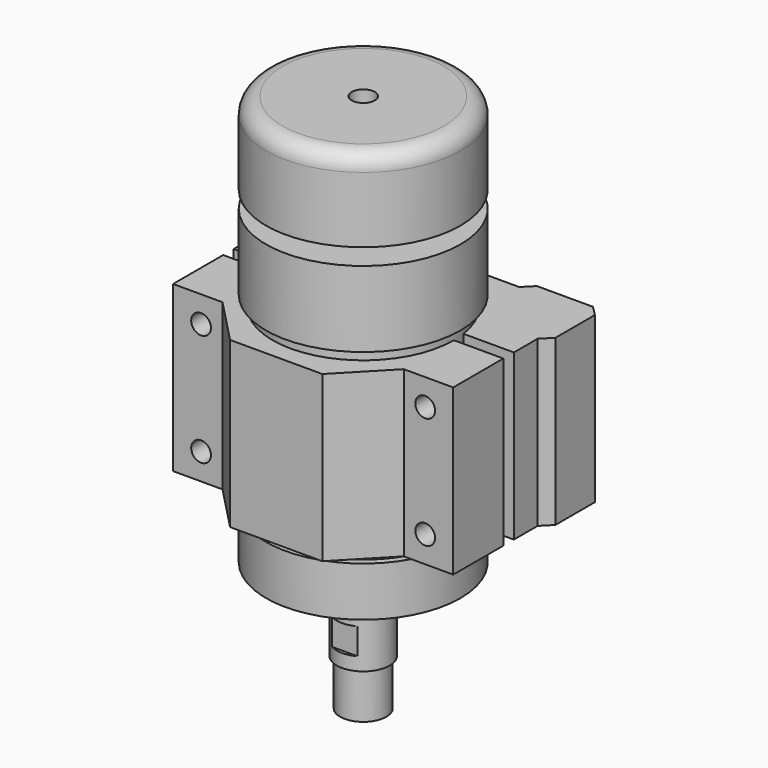
from build123d import *

# Parameters (mm, degrees)
F1_DEPTH      = 28.25
F2_R          = 29.5
F3_DEPTH      = 23
F4_R          = 29.5
F5_DEPTH      = 15
F6_R          = 12.5
F7_DEPTH      = 2
F8_R          = 3.5
F9_DEPTH      = 20
F9_DEPTH_BACK = 120
F11_R         = 8
F11_R_2       = 3.5
F12_DEPTH     = 20
F13_W         = 5.3180262744
F13_H         = 8
F14_DEPTH     = 5
F15_R         = 7
F15_R_2       = 5
F16_DEPTH     = 14
F18_R         = 3.5
F19_DEPTH     = 20
F20_R         = 29.5
F21_DEPTH     = 1.5
F22_R         = 29.5
F22_R_2       = 27.5
F23_DEPTH     = 25
F24_R         = 5
F25_DEPTH     = 25
F27_D         = 6
F27_2_D       = 6


with BuildPart() as f1:
    # F0 (on Top) → F1 (new body, symmetric)
    with BuildSketch(Plane.XY):
        with BuildLine():
            ThreePointArc((-27.5, 0), (0, -27.5), (27.5, 0))
            ThreePointArc((27.5, 0), (27.4267864716, 2.0053388339), (27.2075357208, 4))
            ThreePointArc((27.2075357208, 4), (0, 27.5), (-27.2075357208, 4))
            ThreePointArc((-27.2075357208, 4), (-27.4267864716, 2.0053388339), (-27.5, 0))
        make_face()
    extrude(amount=F1_DEPTH, both=True)

    # F2 (on face) → F3 (join)
    with BuildSketch(Plane.XY.offset(28.25)):
        Circle(F2_R)
        with BuildLine():
            ThreePointArc((-27.5, 0), (-27.4267864716, 2.0053388339), (-27.2075357208, 4))
            ThreePointArc((-27.2075357208, 4), (0, 27.5), (27.2075357208, 4))
            ThreePointArc((27.2075357208, 4), (27.4267864716, 2.0053388339), (27.5, 0))
            ThreePointArc((27.5, 0), (0, -27.5), (-27.5, 0))
        make_face(mode=Mode.SUBTRACT)
        with BuildLine():
            ThreePointArc((27.2075357208, 4), (0, 27.5), (-27.2075357208, 4))
            ThreePointArc((-27.2075357208, 4), (-27.4267864716, 2.0053388339), (-27.5, 0))
            ThreePointArc((-27.5, 0), (0, -27.5), (27.5, 0))
            ThreePointArc((27.5, 0), (27.4267864716, 2.0053388339), (27.2075357208, 4))
        make_face()
    extrude(amount=F3_DEPTH)

    # F4 (on face) → F5 (join)
    with BuildSketch(Plane(origin=(0, 0, -28.25), x_dir=(1, 0, 0), z_dir=(0, 0, -1))):
        Circle(F4_R)
        with BuildLine():
            ThreePointArc((-27.2075357208, -4), (-27.4267864716, -2.0053388339), (-27.5, 0))
            ThreePointArc((-27.5, 0), (0, 27.5), (27.5, 0))
            ThreePointArc((27.5, 0), (27.4267864716, -2.0053388339), (27.2075357208, -4))
            ThreePointArc((27.2075357208, -4), (0, -27.5), (-27.2075357208, -4))
        make_face(mode=Mode.SUBTRACT)
        with BuildLine():
            ThreePointArc((27.5, 0), (0, 27.5), (-27.5, 0))
            ThreePointArc((-27.5, 0), (-27.4267864716, -2.0053388339), (-27.2075357208, -4))
            ThreePointArc((-27.2075357208, -4), (0, -27.5), (27.2075357208, -4))
            ThreePointArc((27.2075357208, -4), (27.4267864716, -2.0053388339), (27.5, 0))
        make_face()
    extrude(amount=F5_DEPTH)

    # F6 (on face) → F7 (join)
    with BuildSketch(Plane(origin=(0, 0, -43.25), x_dir=(1, 0, 0), z_dir=(0, 0, -1))):
        Circle(F6_R)
    extrude(amount=F7_DEPTH)


with BuildPart() as f9:
    # F8 (on face) → F9 (new body, two sides)
    with BuildSketch(Plane(origin=(0, 0, -45.25), x_dir=(1, 0, 0), z_dir=(0, 0, -1))) as f9_sk:
        Circle(F8_R)
    extrude(amount=F9_DEPTH)
    extrude(f9_sk.sketch, amount=-F9_DEPTH_BACK)

    # F11 (on offset) → F12 (join)
    with BuildSketch(Plane(origin=(0, 0, -48.25), x_dir=(1, 0, 0), z_dir=(0, 0, -1))):
        Circle(F11_R)
        Circle(F11_R_2, mode=Mode.SUBTRACT)
    extrude(amount=F12_DEPTH)

    # F13 (on Right) → F14 (cut, symmetric)
    with BuildSketch(Plane.YZ):
        with Locations((9.6590131372, -60.25)):
            Rectangle(F13_W, F13_H)
        with Locations((-9.6590131372, -60.25)):
            Rectangle(F13_W, F13_H)
    extrude(amount=F14_DEPTH, both=True, mode=Mode.SUBTRACT)

    # F15 (on face) → F16 (join)
    with BuildSketch(Plane(origin=(0, 0, -68.25), x_dir=(1, 0, 0), z_dir=(0, 0, -1))):
        Circle(F15_R)
        Circle(F15_R_2, mode=Mode.SUBTRACT)
    extrude(amount=F16_DEPTH)

    # F18 (on offset) → F19 (join)
    with BuildSketch(Plane.XY.offset(61.25)):
        with BuildLine():
            Line((-0.5, -5.4772255751), (-0.5, -29.1325048873))
            Line((-0.5, -29.1325048873), (0.5, -29.1325048873))
            Line((0.5, -29.1325048873), (0.5, -5.4772255751))
            ThreePointArc((0.5, -5.4772255751), (1.6995934691, -5.2308108396), (2.8149239193, -4.7250611984))
            Line((2.8149239193, -4.7250611984), (16.7191482379, -23.8625841687))
            Line((16.7191482379, -23.8625841687), (17.5281652323, -23.2747989164))
            Line((17.5281652323, -23.2747989164), (3.6239409137, -4.1372759461))
            ThreePointArc((3.6239409137, -4.1372759461), (4.4495934691, -3.2328188876), (5.0546425772, -2.1680840429))
            Line((5.0546425772, -2.1680840429), (27.5521501119, -9.477967357))
            Line((27.5521501119, -9.477967357), (27.8611671063, -8.5269108407))
            Line((27.8611671063, -8.5269108407), (5.3636595716, -1.2170275266))
            ThreePointArc((5.3636595716, -1.2170275266), (5.5, 0), (5.3636595716, 1.2170275266))
            Line((5.3636595716, 1.2170275266), (27.8611671063, 8.5269108407))
            Line((27.8611671063, 8.5269108407), (27.5521501119, 9.477967357))
            Line((27.5521501119, 9.477967357), (5.0546425772, 2.1680840429))
            ThreePointArc((5.0546425772, 2.1680840429), (4.4495934691, 3.2328188876), (3.6239409137, 4.1372759461))
            Line((3.6239409137, 4.1372759461), (17.5281652323, 23.2747989164))
            Line((17.5281652323, 23.2747989164), (16.7191482379, 23.8625841687))
            Line((16.7191482379, 23.8625841687), (2.8149239193, 4.7250611984))
            ThreePointArc((2.8149239193, 4.7250611984), (1.6995934691, 5.2308108396), (0.5, 5.4772255751))
            Line((0.5, 5.4772255751), (0.5, 29.1325048873))
            Line((0.5, 29.1325048873), (-0.5, 29.1325048873))
            Line((-0.5, 29.1325048873), (-0.5, 5.4772255751))
            ThreePointArc((-0.5, 5.4772255751), (-1.6995934691, 5.2308108396), (-2.8149239193, 4.7250611984))
            Line((-2.8149239193, 4.7250611984), (-16.7191482379, 23.8625841687))
            Line((-16.7191482379, 23.8625841687), (-17.5281652323, 23.2747989164))
            Line((-17.5281652323, 23.2747989164), (-3.6239409137, 4.1372759461))
            ThreePointArc((-3.6239409137, 4.1372759461), (-4.4495934691, 3.2328188876), (-5.0546425772, 2.1680840429))
            Line((-5.0546425772, 2.1680840429), (-27.5521501119, 9.477967357))
            Line((-27.5521501119, 9.477967357), (-27.8611671063, 8.5269108407))
            Line((-27.8611671063, 8.5269108407), (-5.3636595716, 1.2170275266))
            ThreePointArc((-5.3636595716, 1.2170275266), (-5.5, 0), (-5.3636595716, -1.2170275266))
            Line((-5.3636595716, -1.2170275266), (-27.8611671063, -8.5269108407))
            Line((-27.8611671063, -8.5269108407), (-27.5521501119, -9.477967357))
            Line((-27.5521501119, -9.477967357), (-5.0546425772, -2.1680840429))
            ThreePointArc((-5.0546425772, -2.1680840429), (-4.4495934691, -3.2328188876), (-3.6239409137, -4.1372759461))
            Line((-3.6239409137, -4.1372759461), (-17.5281652323, -23.2747989164))
            Line((-17.5281652323, -23.2747989164), (-16.7191482379, -23.8625841687))
            Line((-16.7191482379, -23.8625841687), (-2.8149239193, -4.7250611984))
            ThreePointArc((-2.8149239193, -4.7250611984), (-1.6995934691, -5.2308108396), (-0.5, -5.4772255751))
        make_face()
        Circle(F18_R, mode=Mode.SUBTRACT)
    extrude(amount=F19_DEPTH)

    # F20 (on face) → F21 (join)
    with BuildSketch(Plane.XY.offset(81.25)):
        Circle(F20_R)
        with BuildLine():
            ThreePointArc((-0.5, -5.4772255751), (-1.6995934691, -5.2308108396), (-2.8149239193, -4.7250611984))
            Line((-2.8149239193, -4.7250611984), (-16.7191482379, -23.8625841687))
            Line((-16.7191482379, -23.8625841687), (-17.5281652323, -23.2747989164))
            Line((-17.5281652323, -23.2747989164), (-3.6239409137, -4.1372759461))
            ThreePointArc((-3.6239409137, -4.1372759461), (-4.4495934691, -3.2328188876), (-5.0546425772, -2.1680840429))
            Line((-5.0546425772, -2.1680840429), (-27.5521501119, -9.477967357))
            Line((-27.5521501119, -9.477967357), (-27.8611671063, -8.5269108407))
            Line((-27.8611671063, -8.5269108407), (-5.3636595716, -1.2170275266))
            ThreePointArc((-5.3636595716, -1.2170275266), (-5.5, 0), (-5.3636595716, 1.2170275266))
            Line((-5.3636595716, 1.2170275266), (-27.8611671063, 8.5269108407))
            Line((-27.8611671063, 8.5269108407), (-27.5521501119, 9.477967357))
            Line((-27.5521501119, 9.477967357), (-5.0546425772, 2.1680840429))
            ThreePointArc((-5.0546425772, 2.1680840429), (-4.4495934691, 3.2328188876), (-3.6239409137, 4.1372759461))
            Line((-3.6239409137, 4.1372759461), (-17.5281652323, 23.2747989164))
            Line((-17.5281652323, 23.2747989164), (-16.7191482379, 23.8625841687))
            Line((-16.7191482379, 23.8625841687), (-2.8149239193, 4.7250611984))
            ThreePointArc((-2.8149239193, 4.7250611984), (-1.6995934691, 5.2308108396), (-0.5, 5.4772255751))
            Line((-0.5, 5.4772255751), (-0.5, 29.1325048873))
            Line((-0.5, 29.1325048873), (0.5, 29.1325048873))
            Line((0.5, 29.1325048873), (0.5, 5.4772255751))
            ThreePointArc((0.5, 5.4772255751), (1.6995934691, 5.2308108396), (2.8149239193, 4.7250611984))
            Line((2.8149239193, 4.7250611984), (16.7191482379, 23.8625841687))
            Line((16.7191482379, 23.8625841687), (17.5281652323, 23.2747989164))
            Line((17.5281652323, 23.2747989164), (3.6239409137, 4.1372759461))
            ThreePointArc((3.6239409137, 4.1372759461), (4.4495934691, 3.2328188876), (5.0546425772, 2.1680840429))
            Line((5.0546425772, 2.1680840429), (27.5521501119, 9.477967357))
            Line((27.5521501119, 9.477967357), (27.8611671063, 8.5269108407))
            Line((27.8611671063, 8.5269108407), (5.3636595716, 1.2170275266))
            ThreePointArc((5.3636595716, 1.2170275266), (5.5, 0), (5.3636595716, -1.2170275266))
            Line((5.3636595716, -1.2170275266), (27.8611671063, -8.5269108407))
            Line((27.8611671063, -8.5269108407), (27.5521501119, -9.477967357))
            Line((27.5521501119, -9.477967357), (5.0546425772, -2.1680840429))
            ThreePointArc((5.0546425772, -2.1680840429), (4.4495934691, -3.2328188876), (3.6239409137, -4.1372759461))
            Line((3.6239409137, -4.1372759461), (17.5281652323, -23.2747989164))
            Line((17.5281652323, -23.2747989164), (16.7191482379, -23.8625841687))
            Line((16.7191482379, -23.8625841687), (2.8149239193, -4.7250611984))
            ThreePointArc((2.8149239193, -4.7250611984), (1.6995934691, -5.2308108396), (0.5, -5.4772255751))
            Line((0.5, -5.4772255751), (0.5, -29.1325048873))
            Line((0.5, -29.1325048873), (-0.5, -29.1325048873))
            Line((-0.5, -29.1325048873), (-0.5, -5.4772255751))
        make_face(mode=Mode.SUBTRACT)
    extrude(amount=-F21_DEPTH)

    # F22 (on face) → F23 (join)
    with BuildSketch(Plane.XY.offset(81.25)):
        Circle(F22_R)
        with Locations((0.5, 0)):
            Circle(F22_R_2, mode=Mode.SUBTRACT)
    extrude(amount=-F23_DEPTH)

    # F24
    f24_edges = [f9.edges().sort_by_distance(p)[0] for p in [
        (-29.5, 0, 81.25),
    ]]
    fillet(f24_edges, radius=F24_R)


with BuildPart() as f25:
    # F0 (on Top) → F25 (new body, symmetric)
    with BuildSketch(Plane.XY):
        with BuildLine():
            Line((42.5, 0), (27.5, 0))
            ThreePointArc((27.5, 0), (0, -27.5), (-27.5, 0))
            Line((-27.5, 0), (-42.5, 0))
            Line((-42.5, 0), (-42.5, -19))
            Line((-42.5, -19), (-27.5, -19))
            Line((-27.5, -19), (-14, -33))
            Line((-14, -33), (0, -33))
            Line((0, -33), (14, -33))
            Line((14, -33), (27.5, -19))
            Line((27.5, -19), (42.5, -19))
            Line((42.5, -19), (42.5, 0))
        make_face()
    extrude(amount=F25_DEPTH, both=True)

    # F27 (through all)
    with Locations(Plane.XZ.offset(19)):
        with Locations((-34, 17), (-34, -17), (34, 17), (34, -17)):
            Hole(F27_D / 2)


with BuildPart() as f25b:
    # F0 (on Top) → F25, piece 2 (new body, symmetric)
    with BuildSketch(Plane.XY):
        with BuildLine():
            ThreePointArc((-27.2075357208, 4), (0, 27.5), (27.2075357208, 4))
            Line((27.2075357208, 4), (42.5, 4))
            Line((42.5, 4), (42.5, 13))
            Line((42.5, 13), (45.5, 16))
            Line((45.5, 16), (45.5, 31))
            Line((45.5, 31), (42.5, 34))
            Line((42.5, 34), (25.5, 34))
            Line((25.5, 34), (22.5, 31))
            Line((22.5, 31), (10, 31))
            Line((10, 31), (7, 34))
            Line((7, 34), (0, 34))
            Line((0, 34), (-7, 34))
            Line((-7, 34), (-10, 31))
            Line((-10, 31), (-22.5, 31))
            Line((-22.5, 31), (-25.5, 34))
            Line((-25.5, 34), (-42.5, 34))
            Line((-42.5, 34), (-45.5, 31))
            Line((-45.5, 31), (-45.5, 16))
            Line((-45.5, 16), (-42.5, 13))
            Line((-42.5, 13), (-42.5, 4))
            Line((-42.5, 4), (-27.2075357208, 4))
        make_face()
    extrude(amount=F25_DEPTH, both=True)

    # F27#2 (through all)
    with Locations(Plane.XZ.offset(19)):
        with Locations((-34, 17), (-34, -17), (34, 17), (34, -17)):
            Hole(F27_2_D / 2)


solid = Compound([f1.part, f9.part, f25.part, f25b.part])
